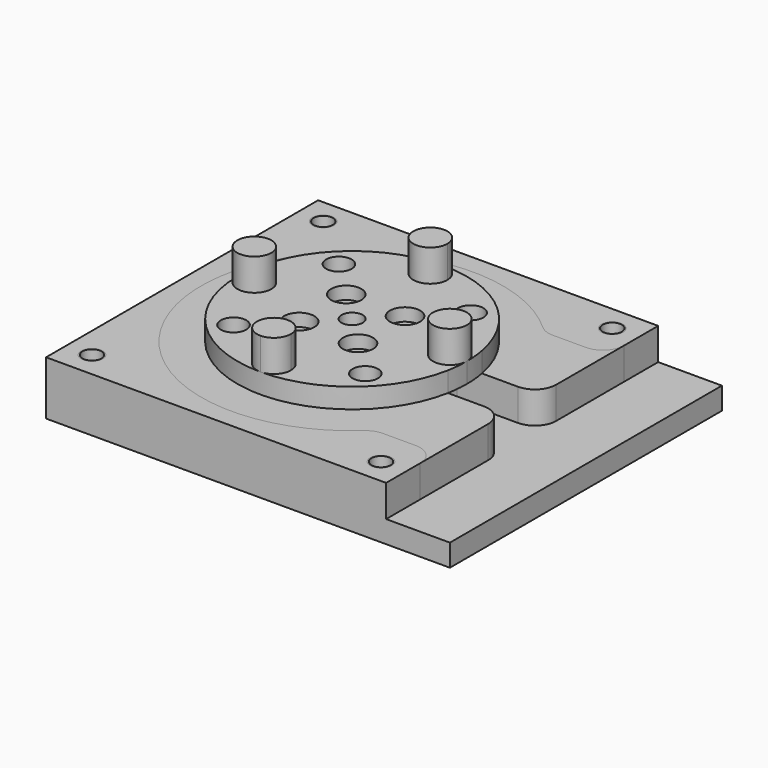
from build123d import *

# Parameters (mm, degrees)
F0_R      = 2.25
F0_R_2    = 3
F0_R_3    = 1.75
F1_DEPTH  = 12.7
F2_R      = 3
F3_DEPTH  = 3
F4_R      = 2.55
F4_R_2    = 27.5
F5_DEPTH  = 12.7
F7_DEPTH  = 7.5
F8_R      = 1.8288
F8_R_2    = 2.5
F8_R_3    = 3
F9_DEPTH  = 4.7
F10_R     = 4
F11_DEPTH = 7.5
F12_R     = 3.556
F12_R_2   = 1.8288
F13_DEPTH = 3


# Not quite as in the source:
# - a length typed as a fraction of an inch, garbled in the dataset ("3 / 203.2 mm" for 3/8 in), is restored
# - a feature names something its author has since deleted; it is built from what else it names


with BuildPart() as f1:
    # F0 (on Top) → F1 (new body)
    with BuildSketch(Plane.XY):
        with BuildLine():
            Line((-40, -40), (40, -40))
            Line((40, -40), (40, -10))
            ThreePointArc((40, -10), (38.5355339059, -6.4644660941), (35, -5))
            Line((35, -5), (20.7123151772, -5))
            ThreePointArc((20.7123151772, -5), (18.0542675119, -5.7650522307), (16.2096379648, -7.8260869565))
            ThreePointArc((16.2096379648, -7.8260869565), (-18, 0), (16.2096379648, 7.8260869565))
            ThreePointArc((16.2096379648, 7.8260869565), (18.0542675119, 5.7650522307), (20.7123151772, 5))
            Line((20.7123151772, 5), (35, 5))
            ThreePointArc((35, 5), (38.5355339059, 6.4644660941), (40, 10))
            Line((40, 10), (40, 40))
            Line((40, 40), (-40, 40))
            Line((-40, 40), (-40, -40))
        make_face()
        with Locations((-34, -34)):
            Circle(F0_R, mode=Mode.SUBTRACT)
        with Locations((-15.5, -15.5)):
            Circle(F0_R_2, mode=Mode.SUBTRACT)
        with Locations((34, -34)):
            Circle(F0_R, mode=Mode.SUBTRACT)
        with Locations((15.5, -15.5)):
            Circle(F0_R_2, mode=Mode.SUBTRACT)
        with Locations((-15.5, 15.5)):
            Circle(F0_R_2, mode=Mode.SUBTRACT)
        with Locations((-34, 34)):
            Circle(F0_R, mode=Mode.SUBTRACT)
        with Locations((15.5, 15.5)):
            Circle(F0_R_2, mode=Mode.SUBTRACT)
        with Locations((34, 34)):
            Circle(F0_R, mode=Mode.SUBTRACT)
        with Locations((-15.5, 15.5)):
            Circle(F0_R_2)
        with Locations((-15.5, 15.5)):
            Circle(F0_R_3, mode=Mode.SUBTRACT)
        with Locations((-15.5, -15.5)):
            Circle(F0_R_2)
        with Locations((-15.5, -15.5)):
            Circle(F0_R_3, mode=Mode.SUBTRACT)
        with Locations((15.5, -15.5)):
            Circle(F0_R_2)
        with Locations((15.5, -15.5)):
            Circle(F0_R_3, mode=Mode.SUBTRACT)
        with Locations((15.5, 15.5)):
            Circle(F0_R_2)
        with Locations((15.5, 15.5)):
            Circle(F0_R_3, mode=Mode.SUBTRACT)
    extrude(amount=F1_DEPTH)

    # F2 (on face) → F3 (cut)
    with BuildSketch(Plane.XY.offset(12.7)):
        with Locations((-15.5, 15.5)):
            Circle(F2_R)
        with Locations((15.5, 15.5)):
            Circle(F2_R)
        with Locations((15.5, -15.5)):
            Circle(F2_R)
        with Locations((-15.5, -15.5)):
            Circle(F2_R)
    extrude(amount=-F3_DEPTH, mode=Mode.SUBTRACT)


with BuildPart() as f5:
    # F4 (on Top) → F5 (new body)
    with BuildSketch(Plane.XY):
        Polygon((40, 40), (-40, 40), (-40, -40), (40, -40), (55, -40), (55, 40), align=None)
        with Locations((-34, -34)):
            Circle(F4_R, mode=Mode.SUBTRACT)
        with Locations((34, -34)):
            Circle(F4_R, mode=Mode.SUBTRACT)
        Circle(F4_R_2, mode=Mode.SUBTRACT)
        with Locations((-34, 34)):
            Circle(F4_R, mode=Mode.SUBTRACT)
        with Locations((34, 34)):
            Circle(F4_R, mode=Mode.SUBTRACT)
    extrude(amount=F5_DEPTH)

    # F6 (on face) → F7 (cut)
    with BuildSketch(Plane.XY.offset(12.7)):
        with BuildLine():
            ThreePointArc((27.2075357208, 25), (25.4073299713, 25.3353178823), (23.8485806936, 26.2962962963))
            ThreePointArc((23.8485806936, 26.2962962963), (-35.5, 0), (23.8485806936, -26.2962962963))
            ThreePointArc((23.8485806936, -26.2962962963), (25.4073299713, -25.3353178823), (27.2075357208, -25))
            Line((27.2075357208, -25), (35, -25))
            ThreePointArc((35, -25), (38.5355339059, -26.4644660941), (40, -30))
            Line((40, -30), (40, -40))
            Line((40, -40), (55, -40))
            Line((55, -40), (55, 40))
            Line((55, 40), (40, 40))
            Line((40, 40), (40, 30))
            ThreePointArc((40, 30), (38.5355339059, 26.4644660941), (35, 25))
            Line((35, 25), (27.2075357208, 25))
        make_face()
    extrude(amount=-F7_DEPTH, mode=Mode.SUBTRACT)


with BuildPart() as f9:
    # F8 (on face) → F9 (new body)
    with BuildSketch(Plane.XY.offset(12.7)):
        with BuildLine():
            ThreePointArc((26.5329983228, -5), (26.8829960637, -2.5108808497), (27, 0))
            ThreePointArc((27, 0), (26.8829960637, 2.5108808497), (26.5329983228, 5))
            Line((26.5329983228, 5), (20.7123151772, 5))
            ThreePointArc((20.7123151772, 5), (18.0542675119, 5.7650522307), (16.2096379648, 7.8260869565))
            ThreePointArc((16.2096379648, 7.8260869565), (-18, 0), (16.2096379648, -7.8260869565))
            ThreePointArc((16.2096379648, -7.8260869565), (18.0542675119, -5.7650522307), (20.7123151772, -5))
            Line((20.7123151772, -5), (26.5329983228, -5))
        make_face()
        with Locations((-6.9147972132, -6.9147972132)):
            Circle(F8_R, mode=Mode.SUBTRACT)
        with Locations((6.9147972132, -6.9147972132)):
            Circle(F8_R, mode=Mode.SUBTRACT)
        with Locations((-6.9147972132, 6.9147972132)):
            Circle(F8_R, mode=Mode.SUBTRACT)
        Circle(F8_R_2, mode=Mode.SUBTRACT)
        with Locations((6.9147972132, 6.9147972132)):
            Circle(F8_R, mode=Mode.SUBTRACT)
        with BuildLine():
            Line((20.7123151772, 5), (26.5329983228, 5))
            ThreePointArc((26.5329983228, 5), (-27, 0), (26.5329983228, -5))
            Line((26.5329983228, -5), (20.7123151772, -5))
            ThreePointArc((20.7123151772, -5), (18.0542675119, -5.7650522307), (16.2096379648, -7.8260869565))
            ThreePointArc((16.2096379648, -7.8260869565), (-18, 0), (16.2096379648, 7.8260869565))
            ThreePointArc((16.2096379648, 7.8260869565), (18.0542675119, 5.7650522307), (20.7123151772, 5))
        make_face()
        with Locations((-15.5, -15.5)):
            Circle(F8_R_3, mode=Mode.SUBTRACT)
        with Locations((15.5, -15.5)):
            Circle(F8_R_3, mode=Mode.SUBTRACT)
        with Locations((-15.5, 15.5)):
            Circle(F8_R_3, mode=Mode.SUBTRACT)
        with Locations((15.5, 15.5)):
            Circle(F8_R_3, mode=Mode.SUBTRACT)
    extrude(amount=F9_DEPTH)

    # F10 (on face) → F11 (join)
    with BuildSketch(Plane.XY.offset(17.4)):
        with BuildLine():
            ThreePointArc((4, 23), (2.8284271082, 25.8284271413), (-4.69e-08, 27))
            ThreePointArc((-4.69e-08, 27), (-2.8284271082, 20.1715728587), (4, 23))
        make_face()
        with BuildLine():
            ThreePointArc((-19, 0), (-22.9999999822, 4), (-27, 3.56e-08))
            ThreePointArc((-27, 3.56e-08), (-23.0000000178, -4), (-19, 0))
        make_face()
        with BuildLine():
            ThreePointArc((4, -23), (-2.8284271362, -20.1715728867), (3.24e-08, -27))
            ThreePointArc((3.24e-08, -27), (2.8284271362, -25.8284271133), (4, -23))
        make_face()
        with Locations((23, 0)):
            Circle(F10_R)
    extrude(amount=F11_DEPTH)

    # F12 (on face) → F13 (cut)
    with BuildSketch(Plane.XY.offset(17.4)):
        with Locations((-6.9147972132, -6.9147972132)):
            Circle(F12_R)
        with Locations((-6.9147972132, -6.9147972132)):
            Circle(F12_R_2, mode=Mode.SUBTRACT)
        with Locations((-6.9147972132, 6.9147972132)):
            Circle(F12_R)
        with Locations((-6.9147972132, 6.9147972132)):
            Circle(F12_R_2, mode=Mode.SUBTRACT)
        with Locations((6.9147972132, 6.9147972132)):
            Circle(F12_R)
        with Locations((6.9147972132, 6.9147972132)):
            Circle(F12_R_2, mode=Mode.SUBTRACT)
        with Locations((6.9147972132, -6.9147972132)):
            Circle(F12_R)
        with Locations((6.9147972132, -6.9147972132)):
            Circle(F12_R_2, mode=Mode.SUBTRACT)
    extrude(amount=-F13_DEPTH, mode=Mode.SUBTRACT)


solid = Compound([f1.part, f5.part, f9.part])
